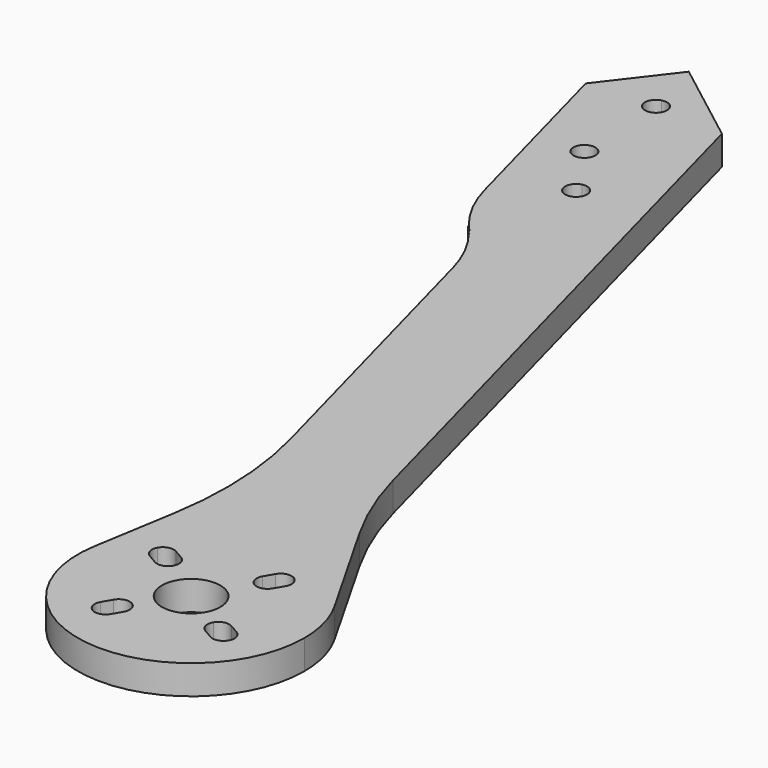
from build123d import *

# Parameters (mm, degrees)
F4_DEPTH = 4
F2_R     = 1.5
F5_DEPTH = 25


with BuildPart() as f4:
    # F3 (on Top) → F4 (new body)
    with BuildSketch(Plane.XY):
        with BuildLine():
            Line((-126.9926666777, -4.22592549), (-132.5, 0))
            Line((-132.5, 0), (-135.7426666777, -4.22592549))
            Line((-135.7426666777, -4.22592549), (-139.4059428918, -9))
            Line((-139.4059428918, -9), (-132.4324272279, -35.0255147652))
            ThreePointArc((-132.4324272279, -35.0255147652), (-130.5316607318, -39.6787820716), (-127.530710333, -43.7111643205))
            Line((-127.530710333, -43.7111643205), (-128.7537766971, -42.4391498951))
            ThreePointArc((-128.7537766971, -42.4391498951), (-125.7528262983, -46.4715321441), (-123.8520598023, -51.1247994505))
            Line((-123.8520598023, -51.1247994505), (-112.6451262464, -92.9496448783))
            ThreePointArc((-112.6451262464, -92.9496448783), (-111.0012337894, -103.4455930684), (-111.6119870301, -114.0519256721))
            Line((-111.6119870301, -114.0519256721), (-113.4985999884, -125.4551601363))
            ThreePointArc((-113.4985999884, -125.4551601363), (-100.9391467421, -112.7279601319), (-84.7430925287, -120.3048535396))
            Line((-84.7430925287, -120.3048535396), (-93.2455614317, -105.4002627224))
            ThreePointArc((-93.2455614317, -105.4002627224), (-96.0587011908, -99.6394303241), (-98.1115817937, -93.5659941915))
            Line((-98.1115817937, -93.5659941915), (-120.7709716444, -9))
            Line((-120.7709716444, -9), (-126.9926666777, -4.22592549))
        make_face()
        with BuildLine():
            ThreePointArc((-82.7064765239, -127.9851719833), (-83.2242795567, -124.0122921667), (-84.7430925287, -120.3048535396))
            ThreePointArc((-84.7430925287, -120.3048535396), (-100.9391467421, -112.7279601319), (-113.4985999884, -125.4551601363))
            ThreePointArc((-113.4985999884, -125.4551601363), (-99.4757452701, -143.4331154338), (-82.7064765239, -127.9851719833))
        make_face()
    extrude(amount=F4_DEPTH)

    # F0 (on Top) + F1 (on Top) + F2 (on Top) → F5 (cut)
    with BuildSketch(Plane.XY):
        with BuildLine():
            ThreePointArc((-101.5723892492, -135.2794656723), (-101.4225386155, -134.1412371047), (-102.1214273549, -133.2304275666))
            ThreePointArc((-102.1214273549, -133.2304275666), (-103.2596559226, -133.0805769329), (-104.1704654606, -133.7794656723))
            Line((-104.1704654606, -133.7794656723), (-104.9204654606, -135.078503778))
            ThreePointArc((-104.9204654606, -135.078503778), (-105.0703160943, -136.2167323456), (-104.3714273549, -137.1275418837))
            ThreePointArc((-104.3714273549, -137.1275418837), (-103.2331987872, -137.2773925174), (-102.3223892492, -136.578503778))
            Line((-102.3223892492, -136.578503778), (-101.5723892492, -135.2794656723))
        make_face()
        with BuildLine():
            ThreePointArc((-94.7423749088, -129.9851719833), (-94.3427732188, -129.0204481637), (-94.2064765239, -127.9851719833))
            ThreePointArc((-94.2064765239, -127.9851719833), (-102.0701798291, -126.9498958029), (-94.7423749088, -129.9851719833))
        make_face()
        with BuildLine():
            Line((-107.4647591496, -123.4853497167), (-106.1657210439, -124.2353497167))
            ThreePointArc((-106.1657210439, -124.2353497167), (-105.0274924763, -124.3852003505), (-104.1166829382, -123.6863116111))
            ThreePointArc((-104.1166829382, -123.6863116111), (-103.9668323045, -122.5480830434), (-104.6657210439, -121.6372735054))
            Line((-104.6657210439, -121.6372735054), (-105.9647591496, -120.8872735054))
            ThreePointArc((-105.9647591496, -120.8872735054), (-107.1029877172, -120.7374228716), (-108.0137972553, -121.4363116111))
            ThreePointArc((-108.0137972553, -121.4363116111), (-108.163647889, -122.5745401787), (-107.4647591496, -123.4853497167))
        make_face()
        with BuildLine():
            Line((-92.523528877, -121.142017922), (-91.773528877, -119.8429798164))
            ThreePointArc((-91.773528877, -119.8429798164), (-91.6236782432, -118.7047512487), (-92.3225669827, -117.7939417107))
            ThreePointArc((-92.3225669827, -117.7939417107), (-93.4607955503, -117.6440910769), (-94.3716050883, -118.3429798164))
            Line((-94.3716050883, -118.3429798164), (-95.1216050883, -119.642017922))
            ThreePointArc((-95.1216050883, -119.642017922), (-95.2714557221, -120.7802464897), (-94.5725669827, -121.6910560277))
            ThreePointArc((-94.5725669827, -121.6910560277), (-93.434338415, -121.8409066615), (-92.523528877, -121.142017922))
        make_face()
        with BuildLine():
            ThreePointArc((-90.5282732936, -130.6861338776), (-91.6665018613, -130.5362832439), (-92.5773113993, -131.2351719833))
            ThreePointArc((-92.5773113993, -131.2351719833), (-92.7271620331, -132.373400551), (-92.0282732936, -133.284210089))
            Line((-92.0282732936, -133.284210089), (-90.729235188, -134.034210089))
            ThreePointArc((-90.729235188, -134.034210089), (-89.5910066203, -134.1840607227), (-88.6801970823, -133.4851719833))
            ThreePointArc((-88.6801970823, -133.4851719833), (-88.5303464485, -132.3469434156), (-89.229235188, -131.4361338776))
            Line((-89.229235188, -131.4361338776), (-90.5282732936, -130.6861338776))
        make_face()
    with BuildSketch(Plane.XY):
        with BuildLine():
            ThreePointArc((-123.2354286469, -28.9777747887), (-123.8222865034, -27.7877447782), (-125.1236572146, -27.5288860492))
            Line((-125.1236572146, -27.5288860492), (-124.3472000793, -30.4266635281))
            ThreePointArc((-124.3472000793, -30.4266635281), (-123.5453986365, -29.8909169322), (-123.2354286469, -28.9777747887))
        make_face()
        with BuildLine():
            Line((-124.3472000793, -30.4266635281), (-125.1236572146, -27.5288860492))
            ThreePointArc((-125.1236572146, -27.5288860492), (-126.1843173864, -29.3660033563), (-124.3472000793, -30.4266635281))
        make_face()
        with BuildLine():
            ThreePointArc((-128.7353333554, -8.45185098), (-129.3221912118, -7.2618209696), (-130.623561923, -7.0029622406))
            Line((-130.623561923, -7.0029622406), (-129.8471047877, -9.9007397195))
            ThreePointArc((-129.8471047877, -9.9007397195), (-129.0453033449, -9.3649931235), (-128.7353333554, -8.45185098))
        make_face()
        with BuildLine():
            Line((-129.8471047877, -9.9007397195), (-130.623561923, -7.0029622406))
            ThreePointArc((-130.623561923, -7.0029622406), (-131.6842220948, -8.8400795477), (-129.8471047877, -9.9007397195))
        make_face()
    with BuildSketch(Plane.XY):
        with Locations((-129.6849733529, -21.3822502318)):
            Circle(F2_R)
    extrude(amount=F5_DEPTH, mode=Mode.SUBTRACT)


solid = f4.part
